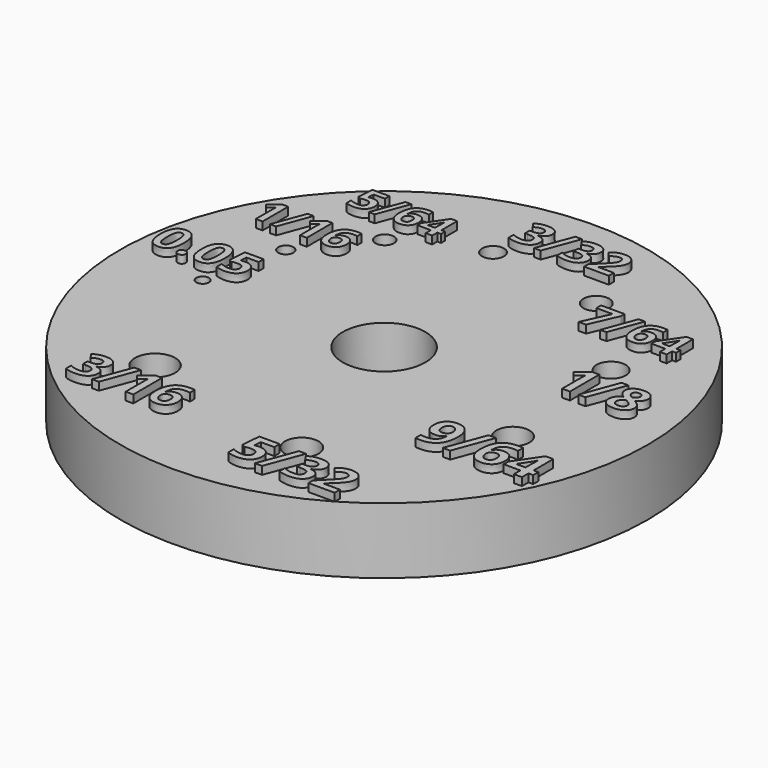
from build123d import *

# Parameters (mm, degrees)
F0_R           = 40
F0_R_2         = 3.05
F0_R_3         = 2.55
F0_R_4         = 2.5
F0_R_5         = 0.95
F0_R_6         = 1.15
F0_R_7         = 1.4
F0_R_8         = 1.65
F0_R_9         = 2.2
F0_R_10        = 1.95
F1_DEPTH       = 10
F2_TEXT_SIZE   = 7.6346746128
F2_TEXT_SIZE_2 = 7.9666135005
F2_TEXT_SIZE_3 = 8.2985601491
F2_TEXT_SIZE_4 = 7.8006456735
F2_TEXT_SIZE_5 = 6.9707916636
F2_TEXT_SIZE_6 = 7.468702582
F2_TEXT_SIZE_7 = 6.6388476019
F2_TEXT_SIZE_8 = 6.8068400853
F2_TEXT_SIZE_9 = 7.2762800199
F3_DEPTH       = 1.2
F5_D           = 6.6
F5_CBORE_D     = 12.5
F5_CBORE_DEPTH = 7


# Not quite as in the source:
# - Text() gives the source's letters only with a copy of the font that has no kerning and outlines rounded to 1/6400 em; it was checked with that copy


with BuildPart() as f1:
    # F0 (on Top) → F1 (new body)
    with BuildSketch(Plane.XY):
        Circle(F0_R)
        with Locations((-18.2520165515, -20.5697324193)):
            Circle(F0_R_2, mode=Mode.SUBTRACT)
        with Locations((8.453965071, -26.1683105029)):
            Circle(F0_R_3, mode=Mode.SUBTRACT)
        with Locations((26.2019374544, -8.3491600557)):
            Circle(F0_R_4, mode=Mode.SUBTRACT)
        with Locations((-27.5, 0)):
            Circle(F0_R_5, mode=Mode.SUBTRACT)
        with Locations((-24.6502482559, 12.1907859027)):
            Circle(F0_R_6, mode=Mode.SUBTRACT)
        with Locations((-17.1222154735, 21.5192875644)):
            Circle(F0_R_7, mode=Mode.SUBTRACT)
        with Locations((-5.1068760575, 27.0216545928)):
            Circle(F0_R_8, mode=Mode.SUBTRACT)
        with Locations((24.6559979776, 12.179152833)):
            Circle(F0_R_9, mode=Mode.SUBTRACT)
        with Locations((12.6071797706, 24.4399062648)):
            Circle(F0_R_10, mode=Mode.SUBTRACT)
    extrude(amount=F1_DEPTH)

    # F2 (on face) → F3 (join)
    with BuildSketch(Plane.XY.offset(10)):
        with Locations((-24.8286705464, -29.8060867935)):
            Text('3/16', F2_TEXT_SIZE, font='Open Sans', font_style=FontStyle.BOLD, text_align=(TextAlign.LEFT, TextAlign.BOTTOM))
        with Locations((3.4926519729, -34.5860570669)):
            Text('5/32', F2_TEXT_SIZE_2, font='Open Sans', font_style=FontStyle.BOLD, text_align=(TextAlign.LEFT, TextAlign.BOTTOM))
        with Locations((18.1910581887, -17.6171660423)):
            Text('9/64', F2_TEXT_SIZE_3, font='Open Sans', font_style=FontStyle.BOLD, text_align=(TextAlign.LEFT, TextAlign.BOTTOM))
        with Locations((22.4930308759, 3.056204645)):
            Text('1/8', F2_TEXT_SIZE_4, font='Open Sans', font_style=FontStyle.BOLD, text_align=(TextAlign.LEFT, TextAlign.BOTTOM))
        with Locations((14.6060809493, 17.6351126283)):
            Text('7/64', F2_TEXT_SIZE_5, font='Open Sans', font_style=FontStyle.BOLD, text_align=(TextAlign.LEFT, TextAlign.BOTTOM))
        with Locations((-4.8722960055, 29.1070397943)):
            Text('3/32', F2_TEXT_SIZE_6, font='Open Sans', font_style=FontStyle.BOLD, text_align=(TextAlign.LEFT, TextAlign.BOTTOM))
        with Locations((-25.4261661321, 24.0880716592)):
            Text('5/64', F2_TEXT_SIZE_7, font='Open Sans', font_style=FontStyle.BOLD, text_align=(TextAlign.LEFT, TextAlign.BOTTOM))
        with Locations((-32.7267423272, 14.3770445138)):
            Text('1/16', F2_TEXT_SIZE_8, font='Open Sans', font_style=FontStyle.BOLD, text_align=(TextAlign.LEFT, TextAlign.BOTTOM))
        with Locations((-37.6276709139, 1.7022348475)):
            Text('0.05', F2_TEXT_SIZE_9, font='Open Sans', font_style=FontStyle.BOLD, text_align=(TextAlign.LEFT, TextAlign.BOTTOM))
    extrude(amount=F3_DEPTH)

    # F5 (through all)
    with Locations(Plane.XY.offset(10)):
        with Locations((0, 0)):
            CounterBoreHole(F5_D / 2, F5_CBORE_D / 2, F5_CBORE_DEPTH)


solid = f1.part
